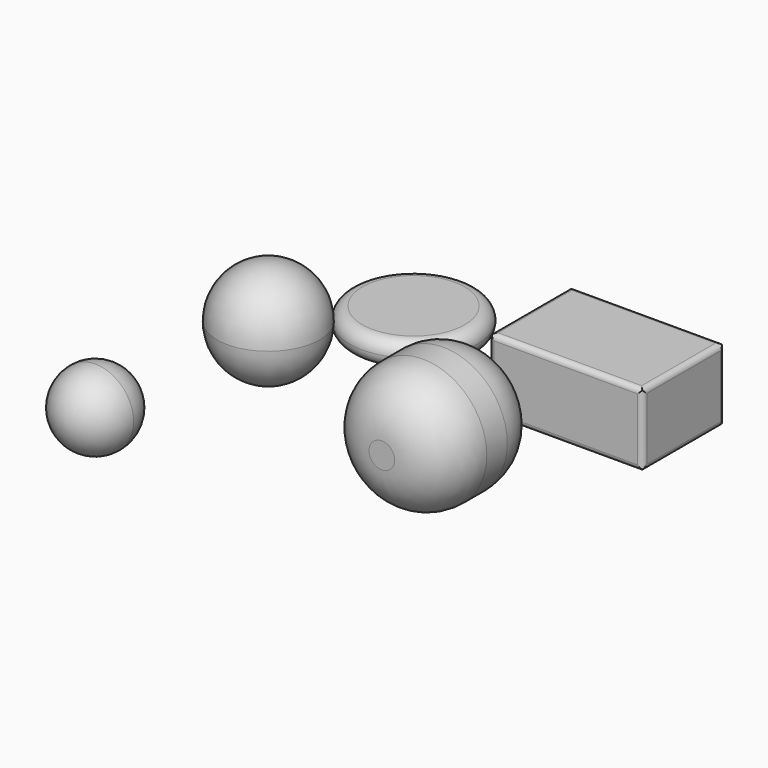
from build123d import *

# Parameters (mm, degrees)
F0_R         = 63.5
F1_DEPTH     = 127
F2_R         = 50.8
F3_R         = 50.8
F4_W         = 101.6
F4_H         = 72.0810802626
F5_DEPTH     = 152.4
F6_R         = 5.08
F7_T1_DEPTH  = 172.72
F7_T3_DEPTH  = 127
F8_T1_DEPTH  = 92.4010802627
F8_T3_DEPTH  = 172.72
F9_T1_DEPTH  = 121.92
F9_T3_DEPTH  = 172.72
F10_T1_DEPTH = 87.3210802627
F11_R        = 63.5
F12_DEPTH    = 25.4
F13_R        = 12.7
F14_R        = 12.69999
F15_R        = 50.8
F16_DEPTH    = 101.6
F17_R        = 50.79999
F18_R        = 38.1
F19_DEPTH    = 76.2
F20_R        = 38.09999


# Not quite as in the source:
# - a fillet or chamfer that OpenCascade refuses, or shapes differently, is made with other operations: its cross-section is extruded or revolved along the edge and cut away or added
# - a fillet or chamfer is up to 0.001 mm smaller than in the source, because OpenCascade refuses the exact size


with BuildPart() as f1:
    # F0 (on Front) → F1 (new body)
    with BuildSketch(Plane.XZ):
        Circle(F0_R)
    extrude(amount=F1_DEPTH)

    # F2
    f2_edges = [f1.edges().sort_by_distance(p)[0] for p in [
        (-63.5, -127, 0),
    ]]
    fillet(f2_edges, radius=F2_R)

    # F3
    f3_edges = [f1.edges().sort_by_distance(p)[0] for p in [
        (-63.5, 0, 0),
    ]]
    fillet(f3_edges, radius=F3_R)


with BuildPart() as f5:
    # F4 (on Right) → F5 (new body)
    with BuildSketch(Plane.YZ):
        with Locations((56.7595242755, 16.5990898386)):
            Rectangle(F4_W, F4_H)
    extrude(amount=F5_DEPTH)

    # F6
    f6_edges = [f5.edges().sort_by_distance(p)[0] for p in [
        (152.4, 56.759524, 52.63963),
        (152.4, 5.959524, 16.59909),
        (152.4, 56.759524, -19.44145),
        (152.4, 107.559524, 16.59909),
    ]]
    fillet(f6_edges, radius=F6_R)

    # F7: fillet of radius 5.08 on 4 edges, made by hand

    # F7_s2 → F7_t1 (cut)
    with BuildSketch(Plane.YZ.offset(-12.7)):
        with BuildLine():
            ThreePointArc((102.4795242755, 52.6396299699), (106.071626724, 51.1517324183), (107.5595242755, 47.5596299699))
            Line((107.5595242755, 47.5596299699), (107.5595242755, 52.6396299699))
            Line((107.5595242755, 52.6396299699), (102.4795242755, 52.6396299699))
        make_face()
        with BuildLine():
            ThreePointArc((11.0395242755, 52.6396299699), (7.4474218271, 51.1517324183), (5.9595242755, 47.5596299699))
            Line((5.9595242755, 47.5596299699), (5.9595242755, 52.6396299699))
            Line((5.9595242755, 52.6396299699), (11.0395242755, 52.6396299699))
        make_face()
    extrude(amount=F7_T1_DEPTH, mode=Mode.SUBTRACT)

    # F7_s4 → F7_t3 (cut)
    with BuildSketch(Plane.XZ.offset(-120.2595242755)):
        with BuildLine():
            ThreePointArc((5.08, 52.6396299699), (1.4878975516, 51.1517324183), (0, 47.5596299699))
            Line((0, 47.5596299699), (0, 52.6396299699))
            Line((0, 52.6396299699), (5.08, 52.6396299699))
        make_face()
    extrude(amount=F7_T3_DEPTH, mode=Mode.SUBTRACT)

    # F8: fillet of radius 5.08 on 4 edges, made by hand

    # F8_s2 → F8_t1 (cut)
    with BuildSketch(Plane.XY.offset(-32.1414502928)):
        with BuildLine():
            ThreePointArc((0, 11.0395242755), (1.4878975516, 7.4474218271), (5.08, 5.9595242755))
            Line((5.08, 5.9595242755), (0, 5.9595242755))
            Line((0, 5.9595242755), (0, 11.0395242755))
        make_face()
    extrude(amount=F8_T1_DEPTH, mode=Mode.SUBTRACT)

    # F8_s4 → F8_t3 (cut)
    with BuildSketch(Plane.YZ.offset(-12.7)):
        with BuildLine():
            ThreePointArc((5.9595242755, -14.3614502928), (7.4474218271, -17.9535527412), (11.0395242755, -19.4414502928))
            Line((11.0395242755, -19.4414502928), (5.9595242755, -19.4414502928))
            Line((5.9595242755, -19.4414502928), (5.9595242755, -14.3614502928))
        make_face()
    extrude(amount=F8_T3_DEPTH, mode=Mode.SUBTRACT)

    # F9: fillet of radius 5.08 on 4 edges, made by hand

    # F9_s2 → F9_t1 (cut)
    with BuildSketch(Plane.XZ.offset(-120.2595242755)):
        with BuildLine():
            ThreePointArc((0, -14.3614502928), (1.4878975516, -17.9535527412), (5.08, -19.4414502928))
            Line((5.08, -19.4414502928), (0, -19.4414502928))
            Line((0, -19.4414502928), (0, -14.3614502928))
        make_face()
    extrude(amount=F9_T1_DEPTH, mode=Mode.SUBTRACT)

    # F9_s4 → F9_t3 (cut)
    with BuildSketch(Plane.YZ.offset(-12.7)):
        with BuildLine():
            ThreePointArc((107.5595242755, -14.3614502928), (106.071626724, -17.9535527412), (102.4795242755, -19.4414502928))
            Line((102.4795242755, -19.4414502928), (107.5595242755, -19.4414502928))
            Line((107.5595242755, -19.4414502928), (107.5595242755, -14.3614502928))
        make_face()
    extrude(amount=F9_T3_DEPTH, mode=Mode.SUBTRACT)

    # F10: fillet of radius 5.08 on 4 edges, made by hand

    # F10_s2 → F10_t1 (cut)
    with BuildSketch(Plane.XY.offset(-27.0614502928)):
        with BuildLine():
            ThreePointArc((0, 102.4795242755), (1.4878975516, 106.071626724), (5.08, 107.5595242755))
            Line((5.08, 107.5595242755), (0, 107.5595242755))
            Line((0, 107.5595242755), (0, 102.4795242755))
        make_face()
    extrude(amount=F10_T1_DEPTH, mode=Mode.SUBTRACT)


with BuildPart() as f12:
    # F11 (on Top) → F12 (new body)
    with BuildSketch(Plane.XY):
        with Locations((-107.0993468165, 46.1539439857)):
            Circle(F11_R)
    extrude(amount=F12_DEPTH)

    # F13
    f13_edges = [f12.edges().sort_by_distance(p)[0] for p in [
        (-170.599347, 46.153944, 0),
    ]]
    fillet(f13_edges, radius=F13_R)

    # F14 (radius 12.7 in the source; OpenCascade refuses exactly that, so slightly less here)
    f14_edges = [f12.edges().sort_by_distance(p)[0] for p in [
        (-170.599347, 46.153944, 25.4),
    ]]
    fillet(f14_edges, radius=F14_R)


with BuildPart() as f16:
    # F15 (on Top) → F16 (new body)
    with BuildSketch(Plane.XY):
        with Locations((-148.5488861799, -82.1063965559)):
            Circle(F15_R)
    extrude(amount=F16_DEPTH)

    # F17 (radius 50.8 in the source; OpenCascade refuses exactly that, so slightly less here)
    f17_edges = [f16.edges().sort_by_distance(p)[0] for p in [
        (-199.348886, -82.106397, 101.6),
        (-97.748886, -82.106397, 50.8),
        (-199.348886, -82.106397, 0),
    ]]
    fillet(f17_edges, radius=F17_R)


with BuildPart() as f19:
    # F18 (on Front) → F19 (new body)
    with BuildSketch(Plane.XZ):
        with Locations((-355.5001616478, -110.0420281291)):
            Circle(F18_R)
    extrude(amount=F19_DEPTH)

    # F20 (radius 38.1 in the source; OpenCascade refuses exactly that, so slightly less here)
    f20_edges = [f19.edges().sort_by_distance(p)[0] for p in [
        (-393.600162, -76.2, -110.042028),
        (-317.400162, -38.1, -110.042028),
        (-393.600162, 0, -110.042028),
    ]]
    fillet(f20_edges, radius=F20_R)


solid = Compound([f1.part, f5.part, f12.part, f16.part, f19.part])
